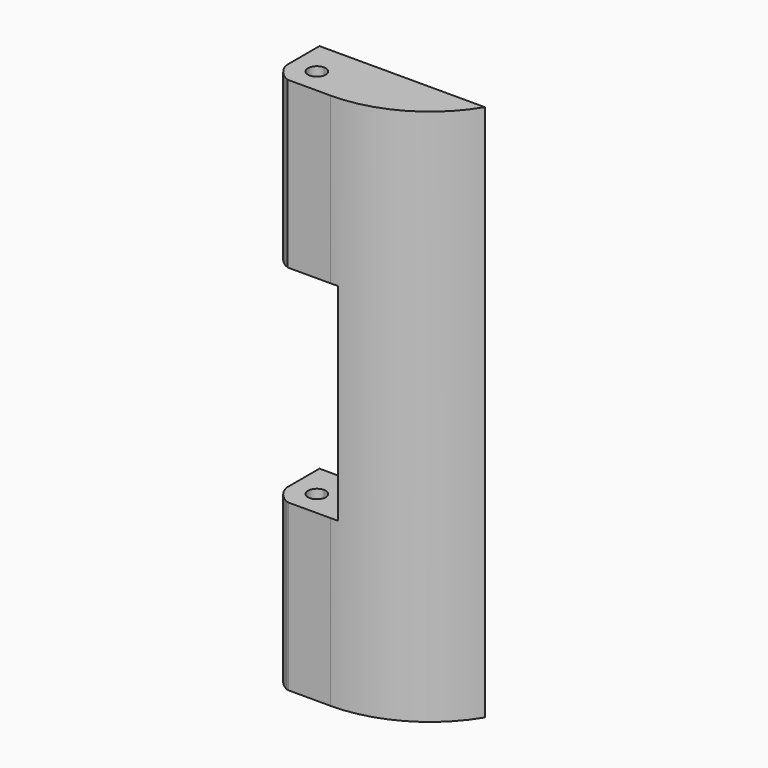
from build123d import *

# Parameters (mm, degrees)
F0_W        = 24
F0_H        = 14.5
F1_DEPTH    = 130
F2_DEPTH    = 130
F3_DEPTH    = 90
F4_DEPTH    = 40
F5_R        = 1
F6_T1_DEPTH = 258.4279953904


# Not quite as in the source:
# - a fillet or chamfer that OpenCascade refuses, or shapes differently, is made with other operations: its cross-section is extruded or revolved along the edge and cut away or added


with BuildPart() as f1:
    # F0 (on Top) → F1 (new body)
    with BuildSketch(Plane.XY):
        with Locations((21.9, 1.16)):
            Rectangle(F0_W, F0_H)
    extrude(amount=F1_DEPTH)

    # F0 (on Top) → F2 (join)
    with BuildSketch(Plane.XY):
        with BuildLine():
            Line((9.9, 8.41), (6.1, 8.41))
            Line((6.1, 8.41), (6.1, -1.59))
            ThreePointArc((6.1, -1.59), (4.7073896383, -4.2954889128), (2.25, -6.09))
            Line((2.25, -6.09), (9.9, -6.09))
            Line((9.9, -6.09), (9.9, 8.41))
        make_face()
        with BuildLine():
            Line((6.1, -1.59), (6.1, 8.41))
            Line((6.1, 8.41), (0, 8.41))
            Line((0, 8.41), (0, 2.15))
            ThreePointArc((0, 2.15), (1.5202795796, 1.5202795796), (2.15, 0))
            ThreePointArc((2.15, 0), (1.5202795796, -1.5202795796), (0, -2.15))
            Line((0, -2.15), (0, -6.09))
            Line((0, -6.09), (2.25, -6.09))
            ThreePointArc((2.25, -6.09), (4.7073896383, -4.2954889128), (6.1, -1.59))
        make_face()
        with BuildLine():
            Line((0, 2.15), (0, 8.41))
            Line((0, 8.41), (-6.1, 8.41))
            Line((-6.1, 8.41), (-6.1, -1.59))
            ThreePointArc((-6.1, -1.59), (-4.7073896383, -4.2954889128), (-2.25, -6.09))
            Line((-2.25, -6.09), (0, -6.09))
            Line((0, -6.09), (0, -2.15))
            ThreePointArc((0, -2.15), (-2.15, 0), (0, 2.15))
        make_face()
    extrude(amount=F2_DEPTH)

    # F0 (on Top) → F3 (cut)
    with BuildSketch(Plane.XY):
        with BuildLine():
            Line((9.9, 8.41), (6.1, 8.41))
            Line((6.1, 8.41), (6.1, -1.59))
            ThreePointArc((6.1, -1.59), (4.7073896383, -4.2954889128), (2.25, -6.09))
            Line((2.25, -6.09), (9.9, -6.09))
            Line((9.9, -6.09), (9.9, 8.41))
        make_face()
        with BuildLine():
            Line((6.1, -1.59), (6.1, 8.41))
            Line((6.1, 8.41), (0, 8.41))
            Line((0, 8.41), (0, 2.15))
            ThreePointArc((0, 2.15), (1.5202795796, 1.5202795796), (2.15, 0))
            ThreePointArc((2.15, 0), (1.5202795796, -1.5202795796), (0, -2.15))
            Line((0, -2.15), (0, -6.09))
            Line((0, -6.09), (2.25, -6.09))
            ThreePointArc((2.25, -6.09), (4.7073896383, -4.2954889128), (6.1, -1.59))
        make_face()
        with BuildLine():
            Line((0, 2.15), (0, 8.41))
            Line((0, 8.41), (-6.1, 8.41))
            Line((-6.1, 8.41), (-6.1, -1.59))
            ThreePointArc((-6.1, -1.59), (-4.7073896383, -4.2954889128), (-2.25, -6.09))
            Line((-2.25, -6.09), (0, -6.09))
            Line((0, -6.09), (0, -2.15))
            ThreePointArc((0, -2.15), (-2.15, 0), (0, 2.15))
        make_face()
    extrude(amount=F3_DEPTH, mode=Mode.SUBTRACT)

    # F0 (on Top) → F4 (join)
    with BuildSketch(Plane.XY):
        with BuildLine():
            Line((0, 2.15), (0, 8.41))
            Line((0, 8.41), (-6.1, 8.41))
            Line((-6.1, 8.41), (-6.1, -1.59))
            ThreePointArc((-6.1, -1.59), (-4.7073896383, -4.2954889128), (-2.25, -6.09))
            Line((-2.25, -6.09), (0, -6.09))
            Line((0, -6.09), (0, -2.15))
            ThreePointArc((0, -2.15), (-2.15, 0), (0, 2.15))
        make_face()
        with BuildLine():
            Line((6.1, -1.59), (6.1, 8.41))
            Line((6.1, 8.41), (0, 8.41))
            Line((0, 8.41), (0, 2.15))
            ThreePointArc((0, 2.15), (1.5202795796, 1.5202795796), (2.15, 0))
            ThreePointArc((2.15, 0), (1.5202795796, -1.5202795796), (0, -2.15))
            Line((0, -2.15), (0, -6.09))
            Line((0, -6.09), (2.25, -6.09))
            ThreePointArc((2.25, -6.09), (4.7073896383, -4.2954889128), (6.1, -1.59))
        make_face()
        with BuildLine():
            Line((9.9, 8.41), (6.1, 8.41))
            Line((6.1, 8.41), (6.1, -1.59))
            ThreePointArc((6.1, -1.59), (4.7073896383, -4.2954889128), (2.25, -6.09))
            Line((2.25, -6.09), (9.9, -6.09))
            Line((9.9, -6.09), (9.9, 8.41))
        make_face()
    extrude(amount=F4_DEPTH)

    # F5
    f5_edges = [f1.edges().sort_by_distance(p)[0] for p in [
        (-2.25, -6.09, 20),
    ]]
    fillet(f5_edges, radius=F5_R)

    # F6: fillet of radius 30 on 1 edges, made by hand

    # F6_s2 → F6_t1 (cut)
    with BuildSketch(Plane.XY.offset(-64.2139976952)):
        with BuildLine():
            ThreePointArc((8.2144009219, -6.09), (22.9622821257, -2.2147009552), (33.9, 8.41))
            Line((33.9, 8.41), (33.9, -6.09))
            Line((33.9, -6.09), (8.2144009219, -6.09))
        make_face()
    extrude(amount=F6_T1_DEPTH, mode=Mode.SUBTRACT)


solid = f1.part
